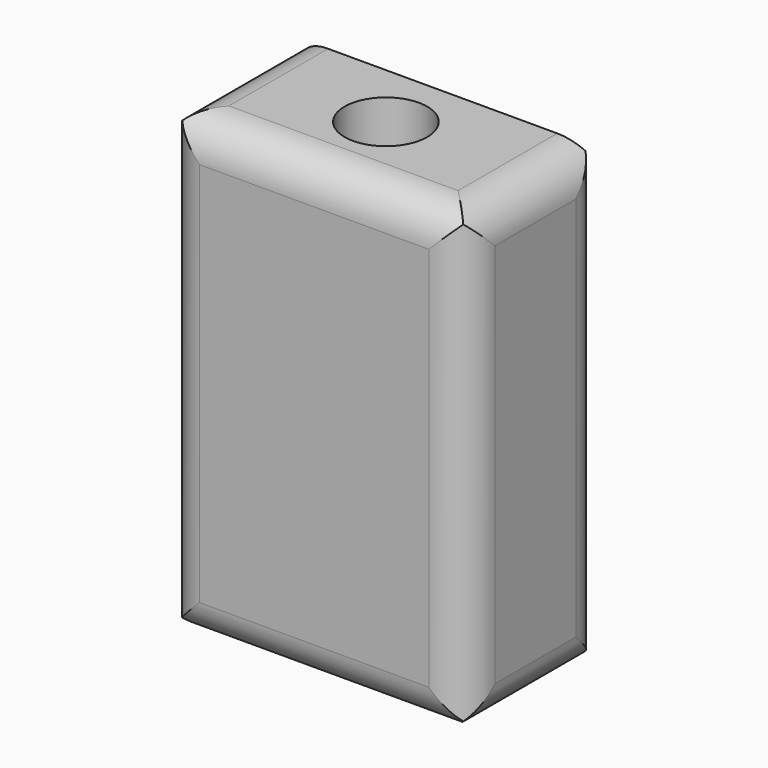
from build123d import *

# Parameters (mm, degrees)
F0_W        = 41.8725572526
F0_H        = 24.7696824372
F1_DEPTH    = 63.5
F3_D        = 11.43
F4_C1_SIZE2 = 5.08
F4_C1_SIZE  = 2.54
F4_C2_SIZE2 = 2.54
F4_C2_SIZE  = 5.08
F4_C3_SIZE2 = 5.08
F4_C3_SIZE  = 2.54
F4_C4_SIZE2 = 2.54
F4_C4_SIZE  = 5.08
F5_R        = 5.08
F6_T1_DEPTH = 42.5496824372
F6_T3_DEPTH = 79.1980633142
F7_T1_DEPTH = 42.5496824372
F7_T3_DEPTH = 79.1980633142


# Not quite as in the source:
# - a fillet or chamfer that OpenCascade refuses, or shapes differently, is made with other operations: its cross-section is extruded or revolved along the edge and cut away or added


with BuildPart() as f1:
    # F0 (on Top) → F1 (new body)
    with BuildSketch(Plane.XY):
        with Locations((20.9362786263, 12.3848412186)):
            Rectangle(F0_W, F0_H)
    extrude(amount=F1_DEPTH)

    # F3 (through all)
    with Locations(Plane.XY.offset(63.5)):
        with Locations((20.6414014101, 12.7780102193)):
            Hole(F3_D / 2)

    # F4: chamfer of 2.54 x 5.08 on 4 edges, made by hand

    # F4_c1
    f4_c1_edges = [f1.edges().sort_by_distance(p)[0] for p in [
        (0, 24.7696824372, 31.75),
    ]]
    f4_c1_side = f1.faces().sort_by_distance((0, 24.7188824372, 31.75))[0]
    chamfer(f4_c1_edges, length=F4_C1_SIZE, length2=F4_C1_SIZE2, reference=f4_c1_side)

    # F4_c2
    f4_c2_edges = [f1.edges().sort_by_distance(p)[0] for p in [
        (41.8725572526, 24.7696824372, 31.75),
    ]]
    f4_c2_side = f1.faces().sort_by_distance((41.8217572526, 24.7696824372, 31.75))[0]
    chamfer(f4_c2_edges, length=F4_C2_SIZE, length2=F4_C2_SIZE2, reference=f4_c2_side)

    # F4_c3
    f4_c3_edges = [f1.edges().sort_by_distance(p)[0] for p in [
        (20.9362786263, 24.7696824372, 0),
    ]]
    f4_c3_side = f1.faces().sort_by_distance((20.9362786263, 24.7188824372, 0))[0]
    chamfer(f4_c3_edges, length=F4_C3_SIZE, length2=F4_C3_SIZE2, reference=f4_c3_side)

    # F4_c4
    f4_c4_edges = [f1.edges().sort_by_distance(p)[0] for p in [
        (20.9362786263, 24.7696824372, 63.5),
    ]]
    f4_c4_side = f1.faces().sort_by_distance((20.9362786263, 24.7696824372, 63.4492))[0]
    chamfer(f4_c4_edges, length=F4_C4_SIZE, length2=F4_C4_SIZE2, reference=f4_c4_side)

    # F5
    f5_edges = [f1.edges().sort_by_distance(p)[0] for p in [
        (0, 0, 31.75),
        (41.872557, 0, 31.75),
        (20.936279, 0, 0),
        (20.936279, 0, 63.5),
    ]]
    fillet(f5_edges, radius=F5_R)

    # F6: fillet of radius 5.08 on 4 edges, made by hand

    # F6_s2 → F6_t1 (cut)
    with BuildSketch(Plane.XZ.offset(-34.9296824372)):
        with BuildLine():
            ThreePointArc((5.08, 0), (1.4878975516, 1.4878975516), (0, 5.08))
            Line((0, 5.08), (0, 0))
            Line((0, 0), (5.08, 0))
        make_face()
        with BuildLine():
            ThreePointArc((5.08, 63.5), (1.4878975516, 62.0121024484), (0, 58.42))
            Line((0, 58.42), (0, 63.5))
            Line((0, 63.5), (5.08, 63.5))
        make_face()
    extrude(amount=F6_T1_DEPTH, mode=Mode.SUBTRACT)

    # F6_s4 → F6_t3 (cut)
    with BuildSketch(Plane.XY.offset(-7.8490316571)):
        with BuildLine():
            ThreePointArc((0, 19.0900697743), (0.7586938936, 21.7607838239), (2.8081549349, 23.6337599046))
            Line((2.8081549349, 23.6337599046), (0, 22.2296824372))
            Line((0, 22.2296824372), (0, 19.0900697743))
        make_face()
    extrude(amount=F6_T3_DEPTH, mode=Mode.SUBTRACT)

    # F7: fillet of radius 5.08 on 4 edges, made by hand

    # F7_s2 → F7_t1 (cut)
    with BuildSketch(Plane.XZ.offset(-34.9296824372)):
        with BuildLine():
            ThreePointArc((41.8725572526, 5.08), (40.3846597011, 1.4878975516), (36.7925572526, 0))
            Line((36.7925572526, 0), (41.8725572526, 0))
            Line((41.8725572526, 0), (41.8725572526, 5.08))
        make_face()
        with BuildLine():
            ThreePointArc((41.8725572526, 58.42), (40.3846597011, 62.0121024484), (36.7925572526, 63.5))
            Line((36.7925572526, 63.5), (41.8725572526, 63.5))
            Line((41.8725572526, 63.5), (41.8725572526, 58.42))
        make_face()
    extrude(amount=F7_T1_DEPTH, mode=Mode.SUBTRACT)

    # F7_s4 → F7_t3 (cut)
    with BuildSketch(Plane.XY.offset(-7.8490316571)):
        with BuildLine():
            ThreePointArc((41.8725572526, 19.0900697743), (41.1138633591, 21.7607838239), (39.0644023178, 23.6337599046))
            Line((39.0644023178, 23.6337599046), (41.8725572526, 22.2296824372))
            Line((41.8725572526, 22.2296824372), (41.8725572526, 19.0900697743))
        make_face()
    extrude(amount=F7_T3_DEPTH, mode=Mode.SUBTRACT)


solid = f1.part
